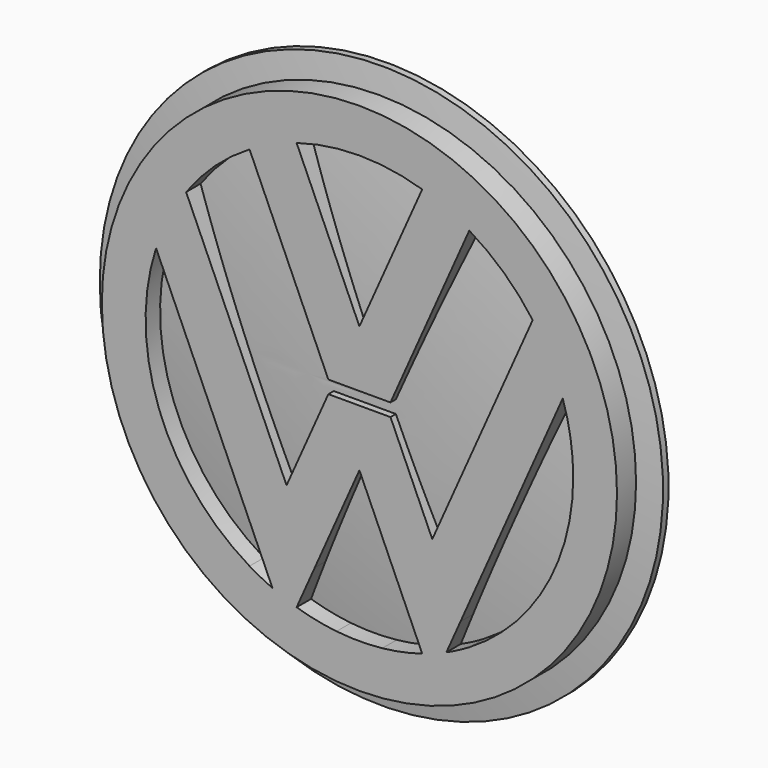
from build123d import *

# Parameters (mm, degrees)
F0_R     = 75
F1_DEPTH = 10


with BuildPart() as f1:
    # F0 (on Front) → F1 (new body)
    with BuildSketch(Plane.XZ):
        Circle(F0_R)
        with BuildLine():
            ThreePointArc((59.2032681394, 19.2363078998), (61.483599202, 9.7380454488), (62.25, 0))
            ThreePointArc((62.25, 0), (54.158206501, -30.6912229895), (31.9865086396, -53.4034246566))
            ThreePointArc((31.9865086396, -53.4034246566), (28.7052557327, -55.2364987424), (25.3193560315, -56.8682047383))
            ThreePointArc((25.3193560315, -56.8682047383), (21.8411530438, -58.2925941584), (18.283326775, -59.5044743027))
            ThreePointArc((18.283326775, -59.5044743027), (12.5301271681, -60.9758838653), (6.6628992551, -61.892392695))
            ThreePointArc((6.6628992551, -61.892392695), (0, -62.25), (-6.6628992551, -61.892392695))
            ThreePointArc((-6.6628992551, -61.892392695), (-12.5301271681, -60.9758838653), (-18.283326775, -59.5044743027))
            ThreePointArc((-18.283326775, -59.5044743027), (-21.8411530438, -58.2925941584), (-25.3193560315, -56.8682047383))
            ThreePointArc((-25.3193560315, -56.8682047383), (-28.7052557327, -55.2364987424), (-31.9865086396, -53.4034246566))
            ThreePointArc((-31.9865086396, -53.4034246566), (-58.2925941584, -21.8411530438), (-59.2032681394, 19.2363078998))
            ThreePointArc((-59.2032681394, 19.2363078998), (-55.5007237058, 28.1909944509), (-50.4533611864, 36.4625951489))
            ThreePointArc((-50.4533611864, 36.4625951489), (-42.0812423811, 45.8719035976), (-31.9865086396, 53.4034246566))
            ThreePointArc((-31.9865086396, 53.4034246566), (-25.3193560315, 56.8682047383), (-18.283326775, 59.5044743027))
            ThreePointArc((-18.283326775, 59.5044743027), (0, 62.25), (18.283326775, 59.5044743027))
            ThreePointArc((18.283326775, 59.5044743027), (25.3193560315, 56.8682047383), (31.9865086396, 53.4034246566))
            ThreePointArc((31.9865086396, 53.4034246566), (42.0812423811, 45.8719035976), (50.4533611864, 36.4625951489))
            ThreePointArc((50.4533611864, 36.4625951489), (55.5007237058, 28.1909944509), (59.2032681394, 19.2363078998))
        make_face(mode=Mode.SUBTRACT)
        with BuildLine():
            Line((29.4242420759, -47.6484797298), (59.2032681394, 19.2363078998))
            ThreePointArc((59.2032681394, 19.2363078998), (55.5007237058, 28.1909944509), (50.4533611864, 36.4625951489))
            Line((50.4533611864, 36.4625951489), (21.2144699871, -29.209029713))
            Line((21.2144699871, -29.209029713), (29.4242420759, -47.6484797298))
        make_face()
        with BuildLine():
            Line((25.3193560315, -56.8682047383), (29.4242420759, -47.6484797298))
            Line((29.4242420759, -47.6484797298), (21.2144699871, -29.209029713))
            Line((21.2144699871, -29.209029713), (13.0046978983, -47.6484797298))
            Line((13.0046978983, -47.6484797298), (18.283326775, -59.5044743027))
            ThreePointArc((18.283326775, -59.5044743027), (21.8411530438, -58.2925941584), (25.3193560315, -56.8682047383))
        make_face()
        with BuildLine():
            Line((9.0445758737, 1.875), (31.9865086396, 53.4034246566))
            ThreePointArc((31.9865086396, 53.4034246566), (25.3193560315, 56.8682047383), (18.283326775, 59.5044743027))
            Line((18.283326775, 59.5044743027), (0, 18.4394500168))
            Line((0, 18.4394500168), (7.3749683038, 1.875))
            Line((7.3749683038, 1.875), (9.0445758737, 1.875))
        make_face()
        Polygon((13.0046978983, -47.6484797298), (21.2144699871, -29.209029713), (9.0445758737, -1.875), (7.3749683038, -1.875), (0, -18.4394500168), align=None)
        with BuildLine():
            Line((0, 18.4394500168), (-18.283326775, 59.5044743027))
            ThreePointArc((-18.283326775, 59.5044743027), (-25.3193560315, 56.8682047383), (-31.9865086396, 53.4034246566))
            Line((-31.9865086396, 53.4034246566), (-9.0445758737, 1.875))
            Line((-9.0445758737, 1.875), (-7.3749683038, 1.875))
            Line((-7.3749683038, 1.875), (0, 18.4394500168))
        make_face()
        Polygon((7.3749683038, 1.875), (0, 18.4394500168), (-7.3749683038, 1.875), align=None)
        Polygon((0, -18.4394500168), (7.3749683038, -1.875), (-7.3749683038, -1.875), align=None)
        Polygon((-13.0046978983, -47.6484797298), (0, -18.4394500168), (-7.3749683038, -1.875), (-9.0445758737, -1.875), (-21.2144699871, -29.209029713), align=None)
        with BuildLine():
            Line((-18.283326775, -59.5044743027), (-13.0046978983, -47.6484797298))
            Line((-13.0046978983, -47.6484797298), (-21.2144699871, -29.209029713))
            Line((-21.2144699871, -29.209029713), (-29.4242420759, -47.6484797298))
            Line((-29.4242420759, -47.6484797298), (-25.3193560315, -56.8682047383))
            ThreePointArc((-25.3193560315, -56.8682047383), (-21.8411530438, -58.2925941584), (-18.283326775, -59.5044743027))
        make_face()
        with BuildLine():
            Line((-21.2144699871, -29.209029713), (-50.4533611864, 36.4625951489))
            ThreePointArc((-50.4533611864, 36.4625951489), (-55.5007237058, 28.1909944509), (-59.2032681394, 19.2363078998))
            Line((-59.2032681394, 19.2363078998), (-29.4242420759, -47.6484797298))
            Line((-29.4242420759, -47.6484797298), (-21.2144699871, -29.209029713))
        make_face()
    extrude(amount=F1_DEPTH)


with BuildPart() as f3:
    # F2 (on Top) → F3 (revolve)
    with BuildSketch(Plane.XY):
        with BuildLine():
            Line((0, -8), (0, 0))
            Line((0, 0), (-82, 0))
            Line((-82, 0), (-82, -2))
            ThreePointArc((-82, -2), (-41.1284722225, -6.7557870405), (0, -8))
        make_face()
    revolve(axis=Axis((0, -4, 0), (0, -1, 0)))


solid = Compound([f1.part, f3.part])
